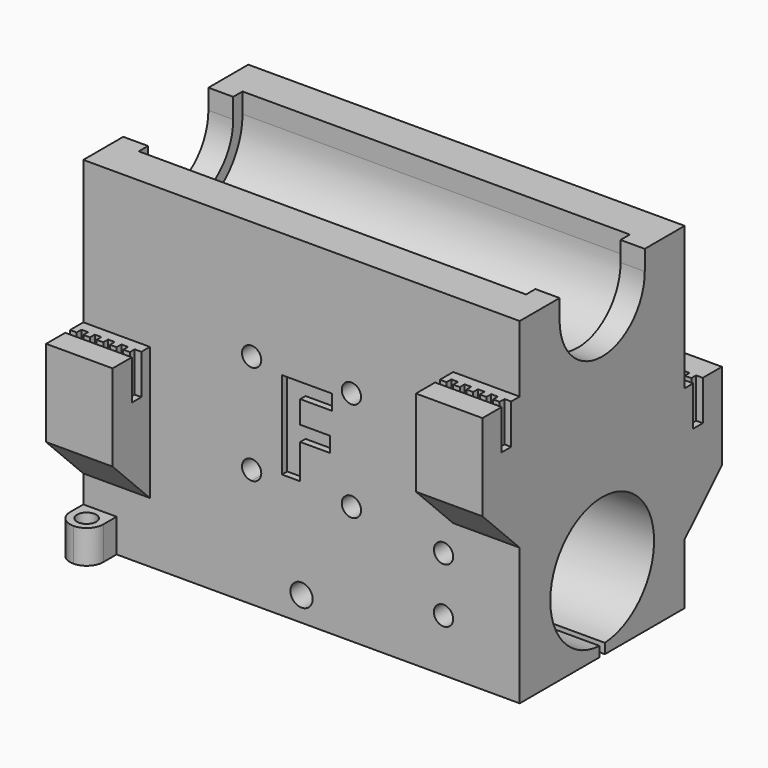
from build123d import *

# Parameters (mm, degrees)
F1_W          = 65.6
F1_H          = 31
F2_DEPTH      = 50.6
F4_DEPTH      = 65.601
F5_DEPTH      = 61.96
F6_DEPTH      = 29.95
F7_DEPTH      = 30.05
F8_DEPTH      = 3.73
F9_W          = 10
F9_H          = 20
F10_DEPTH     = 7
F11_SIZE      = 6.99999
F13_DEPTH     = 6
F15_DEPTH     = 6
F16_W         = 10
F16_H         = 20
F17_DEPTH     = 7
F19_DEPTH     = 6
F21_DEPTH     = 6
F22_SIZE      = 6.99999
F23_R         = 1.45
F23_R_2       = 1.675
F24_DEPTH     = 38.001
F25_R         = 1.45
F26_DEPTH     = 5
F27_TEXT_SIZE = 18.4411155982
F28_DEPTH     = 1
F29_W         = 5
F29_H         = 5
F30_DEPTH     = 5
F32_DEPTH     = 25
F33_R         = 2.49999


# Not quite as in the source:
# - a fillet or chamfer is up to 0.001 mm smaller than in the source, because OpenCascade refuses the exact size
# - Text() gives the source's letters only with a copy of the font that has no kerning and outlines rounded to 1/6400 em; it was checked with that copy


with BuildPart() as f2:
    # F1 (on Top) → F2 (new body)
    with BuildSketch(Plane.XY):
        with Locations((32.8, 15.5)):
            Rectangle(F1_W, F1_H)
    extrude(amount=F2_DEPTH)

    # F3 (on face) → F4 (cut, through all)
    with BuildSketch(Plane(origin=(0, 0, 0), x_dir=(0, -1, 0), z_dir=(-1, 0, 0))):
        with BuildLine():
            Line((-15.5, 15.5999502167), (-9.7236751003, 19.1047164591))
            ThreePointArc((-9.7236751003, 19.1047164591), (-12.4603442198, 20.5140699878), (-15.5, 21))
            Line((-15.5, 21), (-15.5, 15.5999502167))
        make_face()
        with BuildLine():
            Line((-15.5, 15.5999502167), (-15.5, 21))
            ThreePointArc((-15.5, 21), (-18.5396557802, 20.5140699878), (-21.2763248997, 19.1047164591))
            Line((-21.2763248997, 19.1047164591), (-15.5, 15.5999502167))
        make_face()
        with BuildLine():
            Line((-15, 0), (-15, 1.5128289529))
            ThreePointArc((-15, 1.5128289529), (-15.5, 1.5), (-16, 1.5128289529))
            Line((-16, 1.5128289529), (-16, 0))
            Line((-16, 0), (-15.5, 0))
            Line((-15.5, 0), (-15, 0))
        make_face()
        with BuildLine():
            ThreePointArc((-16, 1.5128289529), (-15.5, 1.5), (-15, 1.5128289529))
            Line((-15, 1.5128289529), (-16, 1.5128289529))
        make_face()
        with BuildLine():
            ThreePointArc((-15, 1.5128289529), (-8.4311422422, 4.5348119907), (-5.75, 11.25))
            ThreePointArc((-5.75, 11.25), (-6.7999520756, 15.6513254951), (-9.7236751003, 19.1047164591))
            Line((-9.7236751003, 19.1047164591), (-15.5, 15.5999502167))
            Line((-15.5, 15.5999502167), (-21.2763248997, 19.1047164591))
            ThreePointArc((-21.2763248997, 19.1047164591), (-24.8389876362, 8.4489627045), (-16, 1.5128289529))
            Line((-16, 1.5128289529), (-15, 1.5128289529))
        make_face()
        with BuildLine():
            Line((-7.5, 47.6), (-7.5, 50.6))
            Line((-7.5, 50.6), (-8.0838015129, 50.6))
            ThreePointArc((-8.0838015129, 50.6), (-7.64730658, 49.1281380997), (-7.5, 47.6))
        make_face()
        with BuildLine():
            Line((-22.9161984871, 50.6), (-23.5, 50.6))
            Line((-23.5, 50.6), (-23.5, 47.6))
            ThreePointArc((-23.5, 47.6), (-23.35269342, 49.1281380997), (-22.9161984871, 50.6))
        make_face()
        with BuildLine():
            ThreePointArc((-23.5, 47.6), (-15.5, 39.6), (-7.5, 47.6))
            ThreePointArc((-7.5, 47.6), (-7.64730658, 49.1281380997), (-8.0838015129, 50.6))
            Line((-8.0838015129, 50.6), (-22.9161984871, 50.6))
            ThreePointArc((-22.9161984871, 50.6), (-23.35269342, 49.1281380997), (-23.5, 47.6))
        make_face()
    extrude(amount=-F4_DEPTH, mode=Mode.SUBTRACT)

    # F3 (on face) → F5 (cut)
    with BuildSketch(Plane(origin=(0, 0, 0), x_dir=(0, -1, 0), z_dir=(-1, 0, 0))):
        with BuildLine():
            ThreePointArc((-25.25, 47.6), (-15.5, 37.85), (-5.75, 47.6))
            ThreePointArc((-5.75, 47.6), (-5.8689790349, 49.1185305953), (-6.2230123424, 50.6))
            Line((-6.2230123424, 50.6), (-7.5, 50.6))
            Line((-7.5, 50.6), (-7.5, 47.6))
            ThreePointArc((-7.5, 47.6), (-15.5, 39.6), (-23.5, 47.6))
            Line((-23.5, 47.6), (-23.5, 50.6))
            Line((-23.5, 50.6), (-24.7769876576, 50.6))
            ThreePointArc((-24.7769876576, 50.6), (-25.1310209651, 49.1185305953), (-25.25, 47.6))
        make_face()
        with BuildLine():
            Line((-24.7769876576, 50.6), (-25.25, 50.6))
            Line((-25.25, 50.6), (-25.25, 47.6))
            ThreePointArc((-25.25, 47.6), (-25.1310209651, 49.1185305953), (-24.7769876576, 50.6))
        make_face()
        with BuildLine():
            Line((-5.75, 47.6), (-5.75, 50.6))
            Line((-5.75, 50.6), (-6.2230123424, 50.6))
            ThreePointArc((-6.2230123424, 50.6), (-5.8689790349, 49.1185305953), (-5.75, 47.6))
        make_face()
    extrude(amount=-F5_DEPTH, mode=Mode.SUBTRACT)

    # F3 (on face) → F6 (join)
    with BuildSketch(Plane(origin=(0, 0, 0), x_dir=(0, -1, 0), z_dir=(-1, 0, 0))):
        with BuildLine():
            ThreePointArc((-25.25, 47.6), (-15.5, 37.85), (-5.75, 47.6))
            ThreePointArc((-5.75, 47.6), (-5.8689790349, 49.1185305953), (-6.2230123424, 50.6))
            Line((-6.2230123424, 50.6), (-7.5, 50.6))
            Line((-7.5, 50.6), (-7.5, 47.6))
            ThreePointArc((-7.5, 47.6), (-15.5, 39.6), (-23.5, 47.6))
            Line((-23.5, 47.6), (-23.5, 50.6))
            Line((-23.5, 50.6), (-24.7769876576, 50.6))
            ThreePointArc((-24.7769876576, 50.6), (-25.1310209651, 49.1185305953), (-25.25, 47.6))
        make_face()
        with BuildLine():
            Line((-24.7769876576, 50.6), (-25.25, 50.6))
            Line((-25.25, 50.6), (-25.25, 47.6))
            ThreePointArc((-25.25, 47.6), (-25.1310209651, 49.1185305953), (-24.7769876576, 50.6))
        make_face()
        with BuildLine():
            Line((-5.75, 47.6), (-5.75, 50.6))
            Line((-5.75, 50.6), (-6.2230123424, 50.6))
            ThreePointArc((-6.2230123424, 50.6), (-5.8689790349, 49.1185305953), (-5.75, 47.6))
        make_face()
    extrude(amount=-F6_DEPTH)

    # F3 (on face) → F7 (cut)
    with BuildSketch(Plane(origin=(0, 0, 0), x_dir=(0, -1, 0), z_dir=(-1, 0, 0))):
        with BuildLine():
            ThreePointArc((-25.25, 47.6), (-15.5, 37.85), (-5.75, 47.6))
            ThreePointArc((-5.75, 47.6), (-5.8689790349, 49.1185305953), (-6.2230123424, 50.6))
            Line((-6.2230123424, 50.6), (-7.5, 50.6))
            Line((-7.5, 50.6), (-7.5, 47.6))
            ThreePointArc((-7.5, 47.6), (-15.5, 39.6), (-23.5, 47.6))
            Line((-23.5, 47.6), (-23.5, 50.6))
            Line((-23.5, 50.6), (-24.7769876576, 50.6))
            ThreePointArc((-24.7769876576, 50.6), (-25.1310209651, 49.1185305953), (-25.25, 47.6))
        make_face()
        with BuildLine():
            Line((-24.7769876576, 50.6), (-25.25, 50.6))
            Line((-25.25, 50.6), (-25.25, 47.6))
            ThreePointArc((-25.25, 47.6), (-25.1310209651, 49.1185305953), (-24.7769876576, 50.6))
        make_face()
        with BuildLine():
            Line((-5.75, 47.6), (-5.75, 50.6))
            Line((-5.75, 50.6), (-6.2230123424, 50.6))
            ThreePointArc((-6.2230123424, 50.6), (-5.8689790349, 49.1185305953), (-5.75, 47.6))
        make_face()
    extrude(amount=-F7_DEPTH, mode=Mode.SUBTRACT)

    # F3 (on face) → F8 (join)
    with BuildSketch(Plane(origin=(0, 0, 0), x_dir=(0, -1, 0), z_dir=(-1, 0, 0))):
        with BuildLine():
            ThreePointArc((-25.25, 47.6), (-15.5, 37.85), (-5.75, 47.6))
            ThreePointArc((-5.75, 47.6), (-5.8689790349, 49.1185305953), (-6.2230123424, 50.6))
            Line((-6.2230123424, 50.6), (-7.5, 50.6))
            Line((-7.5, 50.6), (-7.5, 47.6))
            ThreePointArc((-7.5, 47.6), (-15.5, 39.6), (-23.5, 47.6))
            Line((-23.5, 47.6), (-23.5, 50.6))
            Line((-23.5, 50.6), (-24.7769876576, 50.6))
            ThreePointArc((-24.7769876576, 50.6), (-25.1310209651, 49.1185305953), (-25.25, 47.6))
        make_face()
        with BuildLine():
            Line((-24.7769876576, 50.6), (-25.25, 50.6))
            Line((-25.25, 50.6), (-25.25, 47.6))
            ThreePointArc((-25.25, 47.6), (-25.1310209651, 49.1185305953), (-24.7769876576, 50.6))
        make_face()
        with BuildLine():
            Line((-5.75, 47.6), (-5.75, 50.6))
            Line((-5.75, 50.6), (-6.2230123424, 50.6))
            ThreePointArc((-6.2230123424, 50.6), (-5.8689790349, 49.1185305953), (-5.75, 47.6))
        make_face()
    extrude(amount=-F8_DEPTH)

    # F9 (on face) → F10 (join)
    with BuildSketch(Plane.XZ):
        with Locations((5, 19.1)):
            Rectangle(F9_W, F9_H)
        with Locations((60.6, 30.6)):
            Rectangle(F9_W, F9_H)
    extrude(amount=F10_DEPTH)

    # F11 (size 7 in the source; OpenCascade refuses exactly that, so slightly less here)
    f11_edges = [f2.edges().sort_by_distance(p)[0] for p in [
        (5, -7, 9.1),
        (60.6, -7, 20.6),
    ]]
    chamfer(f11_edges, length=F11_SIZE)

    # F12 (on face) → F13 (cut)
    with BuildSketch(Plane.XY.offset(29.1)):
        Polygon((0, -2.5), (0, -3.4), (10, -3.4), (10, -2.5), (10, -1.6), (9, -1.6), (9, -2.5), (8, -2.5), (8, -1.6), (7, -1.6), (7, -2.5), (6, -2.5), (6, -1.6), (5.2958247252, -1.6), (5, -1.6), (5, -2.5), (4, -2.5), (4, -1.6), (3, -1.6), (3, -2.5), (2, -2.5), (2, -1.6), (1, -1.6), (1, -2.5), align=None)
    extrude(amount=-F13_DEPTH, mode=Mode.SUBTRACT)

    # F14 (on face) → F15 (cut)
    with BuildSketch(Plane.XY.offset(40.6)):
        Polygon((55.6, -2.5), (55.6, -3.4), (65.6, -3.4), (65.6, -2.5), (65.6, -1.6), (64.6, -1.6), (64.6, -2.5), (63.6, -2.5), (63.6, -1.6), (62.6, -1.6), (62.6, -2.5), (61.6, -2.5), (61.6, -1.6), (60.8349036932, -1.6), (60.6, -1.6), (60.6, -2.5), (59.6, -2.5), (59.6, -1.6), (58.6, -1.6), (58.6, -2.5), (57.6, -2.5), (57.6, -1.6), (56.6, -1.6), (56.6, -2.5), align=None)
    extrude(amount=-F15_DEPTH, mode=Mode.SUBTRACT)

    # F16 (on face) → F17 (join)
    with BuildSketch(Plane(origin=(0, 31, 0), x_dir=(-1, 0, 0), z_dir=(0, 1, 0))):
        with Locations((-60.6, 19.1)):
            Rectangle(F16_W, F16_H)
        with Locations((-5, 30.6)):
            Rectangle(F16_W, F16_H)
    extrude(amount=F17_DEPTH)

    # F18 (on face) → F19 (cut)
    with BuildSketch(Plane.XY.offset(29.1)):
        Polygon((55.6, 33.5), (55.6, 32.6), (60.6, 32.6), (65.6, 32.6), (65.6, 33.5), (65.6, 34.4), (64.6, 34.4), (64.6, 33.5), (63.6, 33.5), (63.6, 34.4), (62.6, 34.4), (62.6, 33.5), (61.6, 33.5), (61.6, 34.4), (60.6, 34.4), (60.6, 33.5), (59.6, 33.5), (59.6, 34.4), (58.6, 34.4), (58.6, 33.5), (57.6, 33.5), (57.6, 34.4), (56.6, 34.4), (56.6, 33.5), align=None)
    extrude(amount=-F19_DEPTH, mode=Mode.SUBTRACT)

    # F20 (on face) → F21 (cut)
    with BuildSketch(Plane.XY.offset(40.6)):
        Polygon((7, 33.5), (6, 33.5), (6, 34.4), (5, 34.4), (5, 33.5), (4, 33.5), (4, 34.4), (3, 34.4), (3, 33.5), (2, 33.5), (2, 34.4), (1, 34.4), (1, 33.5), (0, 33.5), (0, 32.6), (5, 32.6), (10, 32.6), (10, 33.5), (10, 34.4), (9, 34.4), (9, 33.5), (8, 33.5), (8, 34.4), (7, 34.4), align=None)
    extrude(amount=-F21_DEPTH, mode=Mode.SUBTRACT)

    # F22 (size 7 in the source; OpenCascade refuses exactly that, so slightly less here)
    f22_edges = [f2.edges().sort_by_distance(p)[0] for p in [
        (5, 38, 20.6),
        (60.6, 38, 9.1),
    ]]
    chamfer(f22_edges, length=F22_SIZE)

    # F23 (on face) → F24 (cut, through all)
    with BuildSketch(Plane.XZ):
        with BuildLine():
            ThreePointArc((23.85, 32.8), (25.3, 31.35), (26.75, 32.8))
            ThreePointArc((26.75, 32.8), (25.3, 34.25), (23.85, 32.8))
        make_face()
        with BuildLine():
            ThreePointArc((40.3, 34.25), (39.2746951673, 31.7746951673), (41.75, 32.8))
            ThreePointArc((41.75, 32.8), (41.3253048327, 33.8253048327), (40.3, 34.25))
        make_face()
        with BuildLine():
            ThreePointArc((25.3, 16.35), (26.3253048327, 16.7746951673), (26.75, 17.8))
            ThreePointArc((26.75, 17.8), (24.2746951673, 18.8253048327), (25.3, 16.35))
        make_face()
        with Locations((40.3, 17.8)):
            Circle(F23_R)
        with Locations((32.8, 3.675)):
            Circle(F23_R_2)
        with BuildLine():
            ThreePointArc((41.75, 32.8), (41.3253048327, 33.8253048327), (40.3, 34.25))
            ThreePointArc((40.3, 34.25), (39.2746951673, 31.7746951673), (41.75, 32.8))
        make_face()
        with BuildLine():
            ThreePointArc((26.75, 17.8), (24.2746951673, 18.8253048327), (25.3, 16.35))
            ThreePointArc((25.3, 16.35), (26.3253048327, 16.7746951673), (26.75, 17.8))
        make_face()
    extrude(amount=-F24_DEPTH, mode=Mode.SUBTRACT)

    # F25 (on face) → F26 (cut)
    with BuildSketch(Plane.XZ):
        with Locations((54.15, 16.15)):
            Circle(F25_R)
        with Locations((54.15, 7.9)):
            Circle(F25_R)
    extrude(amount=-F26_DEPTH, mode=Mode.SUBTRACT)

    # F27 (on face) → F28 (cut)
    with BuildSketch(Plane.XZ):
        with Locations((28.1983653734, 18.6611983846)):
            Text('F', F27_TEXT_SIZE, font='Open Sans', font_style=FontStyle.BOLD, text_align=(TextAlign.LEFT, TextAlign.BOTTOM))
    extrude(amount=-F28_DEPTH, mode=Mode.SUBTRACT)

    # F29 (on face) → F30 (join)
    with BuildSketch(Plane.XZ):
        with Locations((2.5, 2.5)):
            Rectangle(F29_W, F29_H)
    extrude(amount=F30_DEPTH)

    # F31 (on face) → F32 (cut)
    with BuildSketch(Plane.XY.offset(5)):
        with BuildLine():
            Line((1.05, -2.5), (3.95, -2.5))
            ThreePointArc((3.95, -2.5), (2.5, -1.05), (1.05, -2.5))
        make_face()
        with BuildLine():
            ThreePointArc((1.05, -2.5), (2.5, -3.95), (3.95, -2.5))
            Line((3.95, -2.5), (1.05, -2.5))
        make_face()
    extrude(amount=-F32_DEPTH, mode=Mode.SUBTRACT)

    # F33 (radius 2.5 in the source; OpenCascade refuses exactly that, so slightly less here)
    f33_edges = [f2.edges().sort_by_distance(p)[0] for p in [
        (0, -5, 2.5),
        (5, -5, 2.5),
    ]]
    fillet(f33_edges, radius=F33_R)


solid = f2.part
